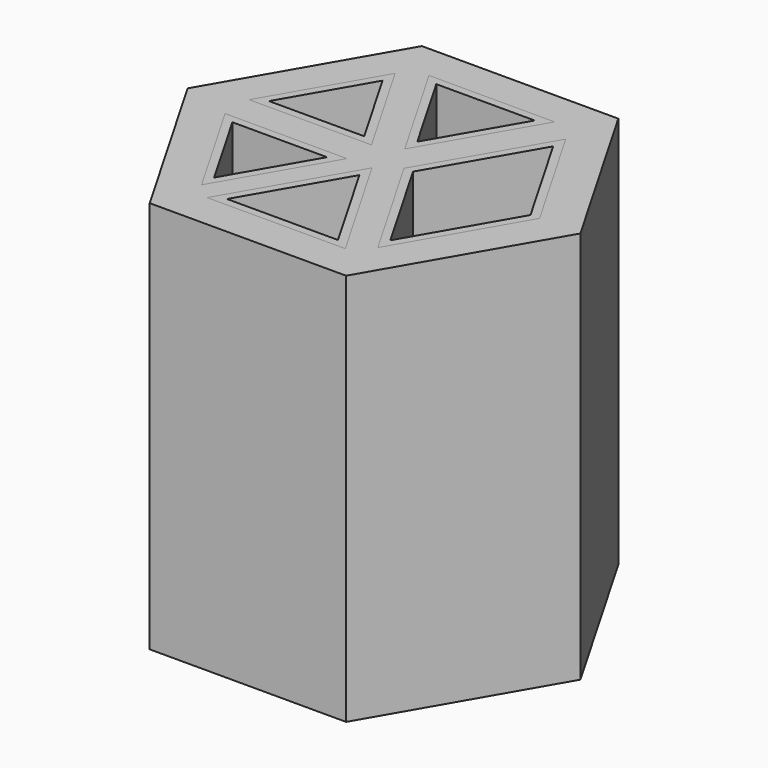
from build123d import *

# Parameters (mm, degrees)
F4_DEPTH = 25.4
F5_DEPTH = 25.4
F6_T     = -0.508
F7_T     = -0.508


# Not quite as in the source:
# - a shell that OpenCascade refuses in one call is made with other operations: the cavity is built on its own and cut out


with BuildPart() as f4:
    # F1 (on Top) → F4 (new body)
    with BuildSketch(Plane.XY):
        Polygon((-6.35, 10.9985226281), (-12.7, 0), (-6.35, -10.9985226281), (6.35, -10.9985226281), (12.7, 0), (6.35, 10.9985226281), align=None)
        Polygon((-5.5598110337, -7.7951700653), (-9.4991829533, -0.9719777506), (-1.620439114, -0.9719777506), align=None, mode=Mode.SUBTRACT)
        Polygon((-4.4690056687, -8.7125226281), (0, -0.9719777506), (4.4690056687, -8.7125226281), align=None, mode=Mode.SUBTRACT)
        Polygon((1.2914098768, 0), (5.675882223, 7.5941288681), (10.0603545693, 0), (5.675882223, -7.5941288681), align=None, mode=Mode.SUBTRACT)
        Polygon((-9.4991829533, 0.9719777506), (-5.5421208235, 7.8258104081), (-1.5850586937, 0.9719777506), align=None, mode=Mode.SUBTRACT)
        Polygon((-4.0627585811, 8.7125226281), (4.0627585811, 8.7125226281), (0, 1.6756183468), align=None, mode=Mode.SUBTRACT)
    extrude(amount=F4_DEPTH)

    # F7
    f7_openings = [f4.faces().sort_by_distance(p)[0] for p in [
        (-0.332472, 0.12346, 0),
    ]]
    offset(amount=F7_T, openings=f7_openings, kind=Kind.INTERSECTION)


with BuildPart() as f5:
    # F3 (on offset) → F5 (new body)
    with BuildSketch(Plane.XY.offset(25.4)):
        Polygon((10.0603545693, 0), (5.675882223, 7.5941288681), (1.2914098768, 0), (5.675882223, -7.5941288681), align=None)
        Polygon((0, 1.6756183468), (4.0627585811, 8.7125226281), (-4.0627585811, 8.7125226281), align=None)
        Polygon((-1.5850586937, 0.9719777506), (-5.5421208235, 7.8258104081), (-9.4991829533, 0.9719777506), align=None)
        Polygon((-1.620439114, -0.9719777506), (-9.4991829533, -0.9719777506), (-5.5598110337, -7.7951700653), align=None)
        Polygon((4.4690056687, -8.7125226281), (0, -0.9719777506), (-4.4690056687, -8.7125226281), align=None)
    extrude(amount=-F5_DEPTH)

    # F6: a shell. OpenCascade refuses it in one call, so the cavity is built on its own and cut out:
    # the body offset inwards by the wall thickness, plus a prism from it out through each open face.
    f6_core = offset(f5.part, amount=F6_T, mode=Mode.PRIVATE)
    f6_exits = [f6_core.faces().sort_by_distance(p)[0] for p in [
        (5.675882, 0, 0.508),
        (0, -6.132341, 0.508),
        (-5.559811, -3.246375, 0.508),
        (-5.542121, 3.256589, 0.508),
        (0, 6.366888, 0.508),
        (-5.542121, 3.256589, 24.892),
        (0, 6.366888, 24.892),
        (5.675882, 0, 24.892),
        (0, -6.132341, 24.892),
        (-5.559811, -3.246375, 24.892),
    ]]
    add(f6_core, mode=Mode.SUBTRACT)
    extrude(f6_exits, amount=-F6_T, mode=Mode.SUBTRACT)


solid = Compound([f4.part, f5.part])
